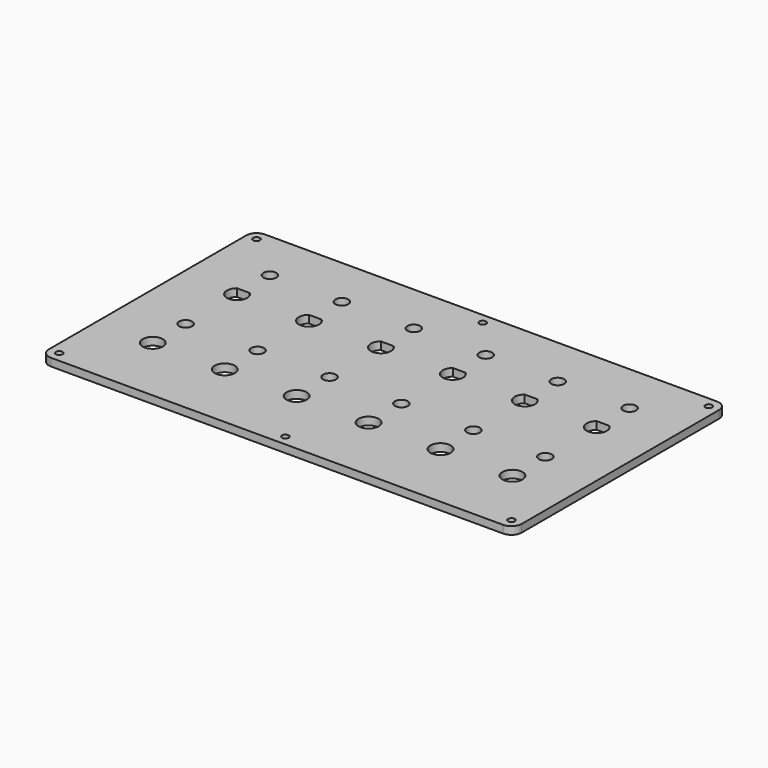
from build123d import *

# Parameters (mm, degrees)
F0_R     = 6.25
F1_DEPTH = 4.7625
F2_D     = 8
F4_D     = 4.1656


# Not quite as in the source:
# - a feature names something its author has since deleted; it is built from what else it names


with BuildPart() as f1:
    # F0 (on Top) → F1 (new body)
    with BuildSketch(Plane.XY):
        with BuildLine():
            Line((163.7876496315, 73.9668203354), (-115.6123503685, 73.9668203354))
            ThreePointArc((-115.6123503685, 73.9668203354), (-120.102478429, 72.1069483959), (-121.9623503685, 67.6168203354))
            Line((-121.9623503685, 67.6168203354), (-121.9623503685, -84.7831796646))
            ThreePointArc((-121.9623503685, -84.7831796646), (-120.102478429, -89.2733077251), (-115.6123503685, -91.1331796646))
            Line((-115.6123503685, -91.1331796646), (163.7876496315, -91.1331796646))
            ThreePointArc((163.7876496315, -91.1331796646), (168.277777692, -89.2733077251), (170.1376496315, -84.7831796646))
            Line((170.1376496315, -84.7831796646), (170.1376496315, 67.6168203354))
            ThreePointArc((170.1376496315, 67.6168203354), (168.277777692, 72.1069483959), (163.7876496315, 73.9668203354))
        make_face()
        with Locations((-87.0373503685, -48.2706796646)):
            Circle(F0_R, mode=Mode.SUBTRACT)
        with Locations((-42.5873503685, -48.2706796646)):
            Circle(F0_R, mode=Mode.SUBTRACT)
        with Locations((1.8626496315, -48.2706796646)):
            Circle(F0_R, mode=Mode.SUBTRACT)
        with Locations((46.3126496315, -48.2706796646)):
            Circle(F0_R, mode=Mode.SUBTRACT)
        with Locations((90.7626496315, -48.2706796646)):
            Circle(F0_R, mode=Mode.SUBTRACT)
        with Locations((135.2126496315, -48.2706796646)):
            Circle(F0_R, mode=Mode.SUBTRACT)
        with BuildLine():
            ThreePointArc((-83.0950236494, 21.6666203354), (-81.3936794889, 19.5022400424), (-80.7873503685, 16.8168203354))
            ThreePointArc((-80.7873503685, 16.8168203354), (-89.7227700755, 11.1731494558), (-90.9796770876, 21.6666203354))
            ThreePointArc((-90.9796770876, 21.6666203354), (-87.0373503685, 23.0668203354), (-83.0950236494, 21.6666203354))
        make_face(mode=Mode.SUBTRACT)
        with BuildLine():
            ThreePointArc((-38.6450236494, 21.6666203354), (-36.9436794889, 19.5022400424), (-36.3373503685, 16.8168203354))
            ThreePointArc((-36.3373503685, 16.8168203354), (-45.2727700755, 11.1731494558), (-46.5296770876, 21.6666203354))
            ThreePointArc((-46.5296770876, 21.6666203354), (-42.5873503685, 23.0668203354), (-38.6450236494, 21.6666203354))
        make_face(mode=Mode.SUBTRACT)
        with BuildLine():
            ThreePointArc((5.8049763506, 21.6666203354), (7.5063205111, 19.5022400424), (8.1126496315, 16.8168203354))
            ThreePointArc((8.1126496315, 16.8168203354), (-0.8227700755, 11.1731494558), (-2.0796770876, 21.6666203354))
            ThreePointArc((-2.0796770876, 21.6666203354), (1.8626496315, 23.0668203354), (5.8049763506, 21.6666203354))
        make_face(mode=Mode.SUBTRACT)
        with BuildLine():
            ThreePointArc((50.2549763506, 21.6666203354), (51.9563205111, 19.5022400424), (52.5626496315, 16.8168203354))
            ThreePointArc((52.5626496315, 16.8168203354), (43.6272299245, 11.1731494558), (42.3703229124, 21.6666203354))
            ThreePointArc((42.3703229124, 21.6666203354), (46.3126496315, 23.0668203354), (50.2549763506, 21.6666203354))
        make_face(mode=Mode.SUBTRACT)
        with BuildLine():
            ThreePointArc((94.7049763506, 21.6666203354), (96.4063205111, 19.5022400424), (97.0126496315, 16.8168203354))
            ThreePointArc((97.0126496315, 16.8168203354), (88.0772299245, 11.1731494558), (86.8203229124, 21.6666203354))
            ThreePointArc((86.8203229124, 21.6666203354), (90.7626496315, 23.0668203354), (94.7049763506, 21.6666203354))
        make_face(mode=Mode.SUBTRACT)
        with BuildLine():
            ThreePointArc((139.1549763506, 21.6666203354), (140.8563205111, 19.5022400424), (141.4626496315, 16.8168203354))
            ThreePointArc((141.4626496315, 16.8168203354), (132.5272299245, 11.1731494558), (131.2703229124, 21.6666203354))
            ThreePointArc((131.2703229124, 21.6666203354), (135.2126496315, 23.0668203354), (139.1549763506, 21.6666203354))
        make_face(mode=Mode.SUBTRACT)
        with BuildLine():
            Line((-46.5296770876, 21.6666203354), (-38.6450236494, 21.6666203354))
            ThreePointArc((-38.6450236494, 21.6666203354), (-42.5873503685, 23.0668203354), (-46.5296770876, 21.6666203354))
        make_face()
        with BuildLine():
            Line((-90.9796770876, 21.6666203354), (-83.0950236494, 21.6666203354))
            ThreePointArc((-83.0950236494, 21.6666203354), (-87.0373503685, 23.0668203354), (-90.9796770876, 21.6666203354))
        make_face()
        with BuildLine():
            Line((131.2703229124, 21.6666203354), (139.1549763506, 21.6666203354))
            ThreePointArc((139.1549763506, 21.6666203354), (135.2126496315, 23.0668203354), (131.2703229124, 21.6666203354))
        make_face()
        with BuildLine():
            Line((42.3703229124, 21.6666203354), (50.2549763506, 21.6666203354))
            ThreePointArc((50.2549763506, 21.6666203354), (46.3126496315, 23.0668203354), (42.3703229124, 21.6666203354))
        make_face()
        with BuildLine():
            Line((-2.0796770876, 21.6666203354), (5.8049763506, 21.6666203354))
            ThreePointArc((5.8049763506, 21.6666203354), (1.8626496315, 23.0668203354), (-2.0796770876, 21.6666203354))
        make_face()
        with BuildLine():
            Line((86.8203229124, 21.6666203354), (94.7049763506, 21.6666203354))
            ThreePointArc((94.7049763506, 21.6666203354), (90.7626496315, 23.0668203354), (86.8203229124, 21.6666203354))
        make_face()
    extrude(amount=F1_DEPTH)

    # F2 (through all)
    with Locations(Plane(origin=(0, 0, 0), x_dir=(1, 0, 0), z_dir=(0, 0, -1))):
        with Locations((46.3126496315, -42.2168203354), (135.2126496315, -42.2168203354), (-87.0373503685, -42.2168203354), (-42.5873503685, -42.2168203354), (1.8626496315, -42.2168203354), (90.7626496315, -42.2168203354), (1.8626496315, 22.8706796646), (-87.0373503685, 22.8706796646), (90.7626496315, 22.8706796646), (-42.5873503685, 22.8706796646), (135.2126496315, 22.8706796646), (46.3126496315, 22.8706796646)):
            Hole(F2_D / 2)

    # F4 (through all)
    with Locations(Plane.XY.offset(4.7625)):
        with Locations((-115.6123503685, 67.6168203354), (163.7876496315, 67.6168203354), (163.7876496315, -84.7831796646), (-115.6123503685, -84.7831796646), (24.0876496315, 67.6168203354), (24.0876496315, -84.7831796646)):
            Hole(F4_D / 2)


solid = f1.part
